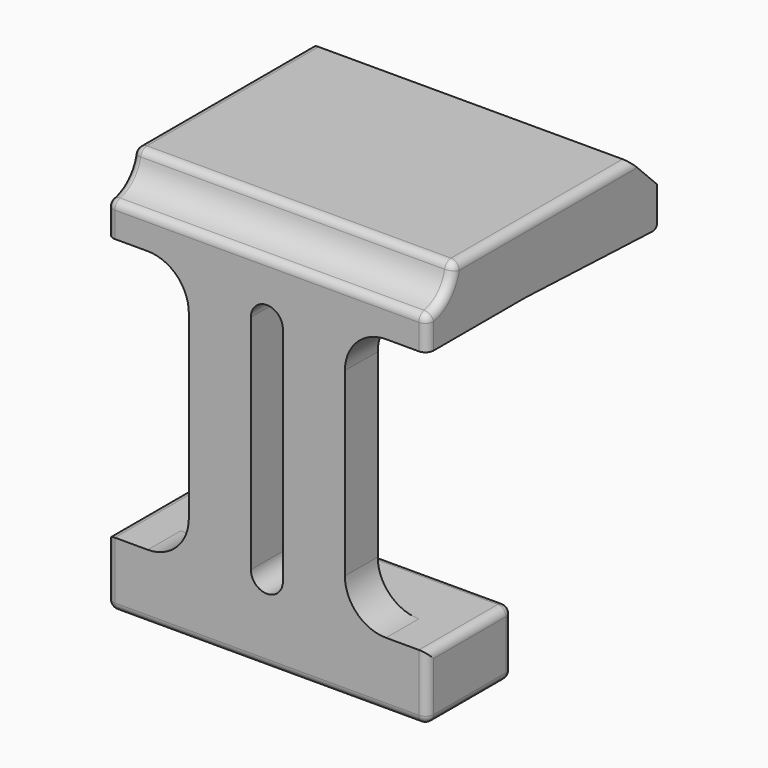
from build123d import *

# Parameters (mm, degrees)
F0_W      = 39
F0_H      = 48
F1_DEPTH  = 5
F2_W      = 10
F2_H      = 32
F3_DEPTH  = 5.001
F4_W      = 39
F4_H      = 8
F5_DEPTH  = 30
F7_DEPTH  = 39
F8_R      = 4
F9_DEPTH  = 39.001
F10_R     = 1
F11_SIZE  = 4
F12_W     = 39
F12_H     = 8
F13_DEPTH = 8
F15_DEPTH = 35.001
F16_R     = 1
F17_R     = 5
F18_R     = 0.6
F19_W     = 7.55
F19_H     = 2.5
F20_DEPTH = 10
F21_SIZE2 = 9.99999
F21_SIZE  = 2.49999
F22_SIZE2 = 2.49999
F22_SIZE  = 9.99999


# Not quite as in the source:
# - a fillet or chamfer is up to 0.001 mm smaller than in the source, because OpenCascade refuses the exact size


with BuildPart() as f1:
    # F0 (on Front) → F1 (new body)
    with BuildSketch(Plane.XZ):
        with Locations((-5.5, 0)):
            Rectangle(F0_W, F0_H)
    extrude(amount=F1_DEPTH)

    # F2 (on face) → F3 (cut, through all)
    with BuildSketch(Plane.XZ.offset(5)):
        with Locations((-20, 0)):
            Rectangle(F2_W, F2_H)
        with Locations((9, 0)):
            Rectangle(F2_W, F2_H)
    extrude(amount=-F3_DEPTH, mode=Mode.SUBTRACT)

    # F4 (on face) → F5 (join)
    with BuildSketch(Plane(origin=(0, 0, 0), x_dir=(-1, 0, 0), z_dir=(0, 1, 0))):
        with Locations((5.5, 20)):
            Rectangle(F4_W, F4_H)
    extrude(amount=F5_DEPTH)

    # F6 (on face) → F7 (join, through all)
    with BuildSketch(Plane.YZ.offset(14)):
        Polygon((30, 16), (10, 16), (30, 15.2), align=None)
    extrude(amount=-F7_DEPTH)

    # F8 (on face) → F9 (cut, through all)
    with BuildSketch(Plane.YZ.offset(14)):
        with Locations((-5, 24)):
            Circle(F8_R)
    extrude(amount=-F9_DEPTH, mode=Mode.SUBTRACT)

    # F10
    f10_edges = [f1.edges().sort_by_distance(p)[0] for p in [
        (-5.5, -1, 24),
        (-5.5, -5, 20),
    ]]
    fillet(f10_edges, radius=F10_R)

    # F11
    f11_edges = [f1.edges().sort_by_distance(p)[0] for p in [
        (-5.5, 30, 24),
    ]]
    chamfer(f11_edges, length=F11_SIZE)

    # F12 (on face) → F13 (join)
    with BuildSketch(Plane(origin=(0, 0, 0), x_dir=(-1, 0, 0), z_dir=(0, 1, 0))):
        with Locations((5.5, -20)):
            Rectangle(F12_W, F12_H)
    extrude(amount=F13_DEPTH)

    # F14 (on face) → F15 (cut, through all)
    with BuildSketch(Plane.XZ.offset(5)):
        with BuildLine():
            Line((-3.55, -14.05), (-3.55, 13))
            ThreePointArc((-3.55, 13), (-5.5, 14.95), (-7.45, 13))
            Line((-7.45, 13), (-7.45, -14.05))
            ThreePointArc((-7.45, -14.05), (-5.5, -16), (-3.55, -14.05))
        make_face()
    extrude(amount=-F15_DEPTH, mode=Mode.SUBTRACT)

    # F16
    f16_edges = [f1.edges().sort_by_distance(p)[0] for p in [
        (-5.5, -4.2, 20.080816),
        (-5.5, -5, -24),
        (-25, -5, -20),
        (14, -5, -20),
        (14, -5, 17.55051),
        (-25, -5, 17.55051),
        (-25, 12.94949, 24),
        (14, 12.94949, 24),
        (14, 1.5, -24),
        (-25, 1.5, -24),
        (-5.5, 8, -16),
        (-5.5, 8, -24),
        (14, 8, -20),
        (-25, 8, -20),
        (-25, 1.5, -16),
        (14, 1.5, -16),
    ]]
    fillet(f16_edges, radius=F16_R)

    # F17
    f17_edges = [f1.edges().sort_by_distance(p)[0] for p in [
        (-15, -2.5, 16),
        (-15, -2.5, -16),
        (4, -2.5, 16),
        (4, -2.5, -16),
    ]]
    fillet(f17_edges, radius=F17_R)

    # F18
    f18_edges = [f1.edges().sort_by_distance(p)[0] for p in [
        (-5.5, 30, 15.2),
    ]]
    fillet(f18_edges, radius=F18_R)

    # F19 (on face) → F20 (join)
    with BuildSketch(Plane(origin=(0, 0, 0), x_dir=(-1, 0, 0), z_dir=(0, 1, 0))):
        with Locations((-0.225, 14.75)):
            Rectangle(F19_W, F19_H)
        with Locations((11.225, 14.75)):
            Rectangle(F19_W, F19_H)
    extrude(amount=F20_DEPTH)

    # F21 (size 2.5 and 10 in the source; OpenCascade refuses exactly that, so slightly less here)
    f21_edges = [f1.edges().sort_by_distance(p)[0] for p in [
        (0.225, 10, 13.5),
    ]]
    f21_side = f1.faces().sort_by_distance((0.225, 10, 14.75))[0]
    chamfer(f21_edges, length=F21_SIZE, length2=F21_SIZE2, reference=f21_side)

    # F22 (size 10 and 2.5 in the source; OpenCascade refuses exactly that, so slightly less here)
    f22_edges = [f1.edges().sort_by_distance(p)[0] for p in [
        (-11.225, 10, 13.5),
    ]]
    f22_side = f1.faces().sort_by_distance((-11.225, 5, 13.5))[0]
    chamfer(f22_edges, length=F22_SIZE, length2=F22_SIZE2, reference=f22_side)


solid = f1.part
